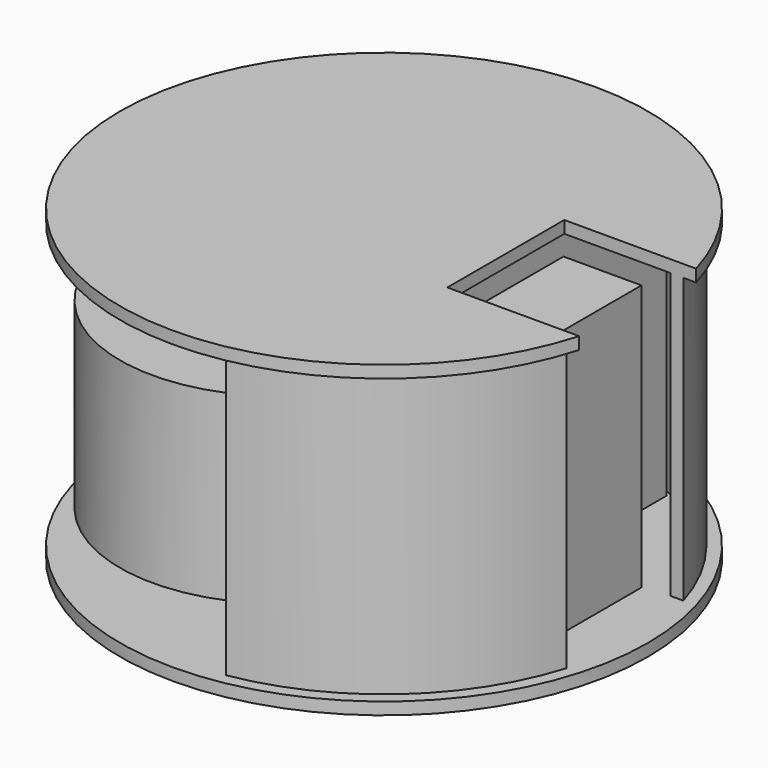
from build123d import *

# Parameters (mm, degrees)
F0_W      = 19.2
F0_H      = 34.5
F1_DEPTH  = 68.5
F2_R      = 65
F2_W      = 3
F2_H      = 5
F3_DEPTH  = 3
F4_R      = 40
F5_DEPTH  = 45
F6_W      = 3
F6_H      = 36
F6_H_2    = 32.1239784062
F7_DEPTH  = 70
F11_DEPTH = 3
F13_DEPTH = 3


# Not quite as in the source:
# - a feature names something its author has since deleted; it is built from what else it names
# - the program builds the solid bodies; features that only make, move or delete a surface that nothing else refers to are left out


with BuildPart() as f1:
    # F0 (on Top) → F1 (new body)
    with BuildSketch(Plane.XY):
        Rectangle(F0_W, F0_H)
    extrude(amount=F1_DEPTH)

    # F2 (on Top) → F3 (join)
    with BuildSketch(Plane.XY):
        with Locations((-40, 0)):
            Circle(F2_R)
        with Locations((-13.5, -12.5)):
            Rectangle(F2_W, F2_H, mode=Mode.SUBTRACT)
        with Locations((-1.5, -19.75)):
            Rectangle(F2_W, F2_H, mode=Mode.SUBTRACT)
        Polygon((-58.5, -4), (-61.5, -4), (-61.5, -1.5), (-64, -1.5), (-64, 1.5), (-61.5, 1.5), (-61.5, 4), (-58.5, 4), (-58.5, 1.5), (-56, 1.5), (-56, -1.5), (-58.5, -1.5), align=None, mode=Mode.SUBTRACT)
        with Locations((-1.5, 19.75)):
            Rectangle(F2_W, F2_H, mode=Mode.SUBTRACT)
        with Locations((-13.5, -12.5)):
            Rectangle(F2_W, F2_H)
    extrude(amount=F3_DEPTH)

    # F4 (on face) → F5 (join)
    with BuildSketch(Plane.XY.offset(3)):
        with Locations((-65, 0)):
            Circle(F4_R)
    extrude(amount=F5_DEPTH)

    # F6 (on face) → F7 (join)
    with BuildSketch(Plane.XY.offset(3)):
        with Locations((-12, 0)):
            Rectangle(F6_W, F6_H)
        with Locations((-12, 34.0619892031)):
            Rectangle(F6_W, F6_H_2)
        with Locations((-12, -34.0619892031)):
            Rectangle(F6_W, F6_H_2)
        with BuildLine():
            Line((19.3295878968, -18), (16.1871871515, -18))
            ThreePointArc((16.1871871515, -18), (-1.2944625099, -44.5295561128), (-30, -58.1463670404))
            Line((-30, -58.1463670404), (-30, -61.1882341631))
            ThreePointArc((-30, -61.1882341631), (0.8405904954, -46.6481100151), (19.3295878968, -18))
        make_face()
        with BuildLine():
            Line((-30, 61.1882341631), (-30, 58.1463670404))
            ThreePointArc((-30, 58.1463670404), (-1.2944625099, 44.5295561128), (16.1871871515, 18))
            Line((16.1871871515, 18), (19.3295878968, 18))
            ThreePointArc((19.3295878968, 18), (0.8405904954, 46.6481100151), (-30, 61.1882341631))
        make_face()
    extrude(amount=F7_DEPTH)

    # F10 (on offset) → F11 (join)
    with BuildSketch(Plane.XY.offset(73)):
        with BuildLine():
            ThreePointArc((22.4579858785, 18), (-105, 0), (22.4579858785, -18))
            Line((22.4579858785, -18), (-10, -18))
            Line((-10, -18), (-10, 18))
            Line((-10, 18), (22.4579858785, 18))
        make_face()
    extrude(amount=F11_DEPTH)

    # F12 (on face) → F13 (join)
    with BuildSketch(Plane(origin=(0, 0, 73), x_dir=(1, 0, 0), z_dir=(0, 0, -1))):
        with BuildLine():
            Line((-13.5, -10.5), (-13.5, -7.5))
            Line((-13.5, -7.5), (-40, -7.5))
            ThreePointArc((-40, -7.5), (-47.5, 0), (-40, 7.5))
            Line((-40, 7.5), (-13.5, 7.5))
            Line((-13.5, 7.5), (-13.5, 10.5))
            Line((-13.5, 10.5), (-40, 10.5))
            ThreePointArc((-40, 10.5), (-50.5, 0), (-40, -10.5))
            Line((-40, -10.5), (-13.5, -10.5))
        make_face()
    extrude(amount=F13_DEPTH)


solid = f1.part
